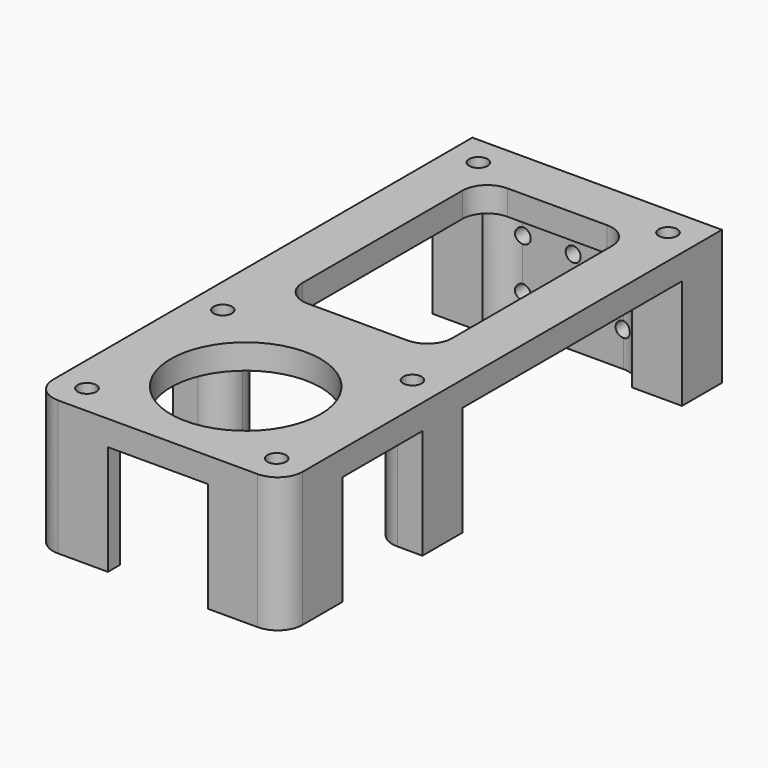
from build123d import *

# Parameters (mm, degrees)
F0_R        = 1.85
F0_R_2      = 15
F0_W        = 10
F0_H        = 10
F1_DEPTH    = 5
F2_DEPTH    = 22
F3_R        = 4.99999
F4_T1_DEPTH = 22
F5_R        = 1.5
F6_DEPTH    = 25


# Not quite as in the source:
# - a fillet or chamfer that OpenCascade refuses, or shapes differently, is made with other operations: its cross-section is extruded or revolved along the edge and cut away or added
# - a fillet or chamfer is up to 0.001 mm smaller than in the source, because OpenCascade refuses the exact size
# - a feature names something its author has since deleted; it is built from what else it names


with BuildPart() as f1:
    # F0 (on Top) → F1 (new body)
    with BuildSketch(Plane.XY):
        with BuildLine():
            Line((0, 15), (0, 0))
            Line((0, 0), (15, 0))
            Line((15, 0), (15, 3))
            ThreePointArc((15, 3), (8.6554793841, 7.8795661534), (5, 15))
            Line((5, 15), (0, 15))
        make_face()
        with Locations((6, 6)):
            Circle(F0_R, mode=Mode.SUBTRACT)
        with BuildLine():
            Line((15, 3), (15, 0))
            Line((15, 0), (35, 0))
            Line((35, 0), (35, 3))
            ThreePointArc((35, 3), (41.3445206159, 7.8795661534), (45, 15))
            Line((45, 15), (50, 15))
            Line((50, 15), (50, 35))
            Line((50, 35), (40, 35))
            Line((40, 35), (40, 45))
            Line((40, 45), (50, 45))
            Line((50, 45), (50, 100))
            Line((50, 100), (40, 100))
            Line((40, 100), (40, 104))
            Line((40, 104), (10, 104))
            Line((10, 104), (10, 100))
            Line((10, 100), (0, 100))
            Line((0, 100), (0, 45))
            Line((0, 45), (10, 45))
            Line((10, 45), (10, 35))
            Line((10, 35), (0, 35))
            Line((0, 35), (0, 15))
            Line((0, 15), (5, 15))
            ThreePointArc((5, 15), (8.6554793841, 7.8795661534), (15, 3))
        make_face()
        with Locations((25, 21.983)):
            Circle(F0_R_2, mode=Mode.SUBTRACT)
        with BuildLine():
            Line((15, 100), (35, 100))
            ThreePointArc((35, 100), (38.5355339059, 98.5355339059), (40, 95))
            Line((40, 95), (40, 55))
            ThreePointArc((40, 55), (38.5355339059, 51.4644660941), (35, 50))
            Line((35, 50), (15, 50))
            ThreePointArc((15, 50), (11.4644660941, 51.4644660941), (10, 55))
            Line((10, 55), (10, 95))
            ThreePointArc((10, 95), (11.4644660941, 98.5355339059), (15, 100))
        make_face(mode=Mode.SUBTRACT)
        with BuildLine():
            Line((35, 3), (35, 0))
            Line((35, 0), (50, 0))
            Line((50, 0), (50, 15))
            Line((50, 15), (45, 15))
            ThreePointArc((45, 15), (41.3445206159, 7.8795661534), (35, 3))
        make_face()
        with Locations((44, 6)):
            Circle(F0_R, mode=Mode.SUBTRACT)
        Polygon((0, 110), (0, 100), (10, 100), (10, 104), (40, 104), (40, 100), (50, 100), (50, 110), align=None)
        with Locations((6, 104)):
            Circle(F0_R, mode=Mode.SUBTRACT)
        with Locations((44, 104)):
            Circle(F0_R, mode=Mode.SUBTRACT)
        with Locations((5, 40)):
            Rectangle(F0_W, F0_H)
        with Locations((6, 40)):
            Circle(F0_R, mode=Mode.SUBTRACT)
        with Locations((45, 40)):
            Rectangle(F0_W, F0_H)
        with Locations((44, 40)):
            Circle(F0_R, mode=Mode.SUBTRACT)
    extrude(amount=F1_DEPTH)

    # F0 (on Top) → F2 (join)
    with BuildSketch(Plane.XY):
        with BuildLine():
            Line((35, 3), (35, 0))
            Line((35, 0), (50, 0))
            Line((50, 0), (50, 15))
            Line((50, 15), (45, 15))
            ThreePointArc((45, 15), (41.3445206159, 7.8795661534), (35, 3))
        make_face()
        with Locations((44, 6)):
            Circle(F0_R, mode=Mode.SUBTRACT)
        with BuildLine():
            Line((0, 15), (0, 0))
            Line((0, 0), (15, 0))
            Line((15, 0), (15, 3))
            ThreePointArc((15, 3), (8.6554793841, 7.8795661534), (5, 15))
            Line((5, 15), (0, 15))
        make_face()
        with Locations((6, 6)):
            Circle(F0_R, mode=Mode.SUBTRACT)
        with Locations((45, 40)):
            Rectangle(F0_W, F0_H)
        with Locations((44, 40)):
            Circle(F0_R, mode=Mode.SUBTRACT)
        with Locations((5, 40)):
            Rectangle(F0_W, F0_H)
        with Locations((6, 40)):
            Circle(F0_R, mode=Mode.SUBTRACT)
        Polygon((0, 110), (0, 100), (10, 100), (10, 104), (40, 104), (40, 100), (50, 100), (50, 110), align=None)
        with Locations((6, 104)):
            Circle(F0_R, mode=Mode.SUBTRACT)
        with Locations((44, 104)):
            Circle(F0_R, mode=Mode.SUBTRACT)
    extrude(amount=-F2_DEPTH)

    # F3 (radius 5 in the source; OpenCascade refuses exactly that, so slightly less here)
    f3_edges = [f1.edges().sort_by_distance(p)[0] for p in [
        (50, 0, -8.5),
        (0, 0, -8.5),
        (40, 35, -11),
        (40, 45, -11),
        (10, 35, -11),
        (10, 45, -11),
    ]]
    fillet(f3_edges, radius=F3_R)

    # F4: fillet of radius 5 on 2 edges, made by hand

    # F4_s2 → F4_t1 (join)
    with BuildSketch(Plane.XY.offset(-22)):
        with BuildLine():
            ThreePointArc((35.1010205144, 104), (38.2632981746, 102.8729833462), (40, 100))
            Line((40, 100), (40, 104))
            Line((40, 104), (35.1010205144, 104))
        make_face()
        with BuildLine():
            ThreePointArc((10, 100), (11.7367018254, 102.8729833462), (14.8989794856, 104))
            Line((14.8989794856, 104), (10, 104))
            Line((10, 104), (10, 100))
        make_face()
    extrude(amount=F4_T1_DEPTH)

    # F5 (on face) → F6 (cut)
    with BuildSketch(Plane(origin=(0, 110, 0), x_dir=(-1, 0, 0), z_dir=(0, 1, 0))):
        with Locations((-35, -15)):
            Circle(F5_R)
        with Locations((-35, -5)):
            Circle(F5_R)
        with Locations((-15, -5)):
            Circle(F5_R)
        with Locations((-15, -15)):
            Circle(F5_R)
        with Locations((-25, -15)):
            Circle(F5_R)
        with Locations((-25, -5)):
            Circle(F5_R)
    extrude(amount=-F6_DEPTH, mode=Mode.SUBTRACT)


solid = f1.part
